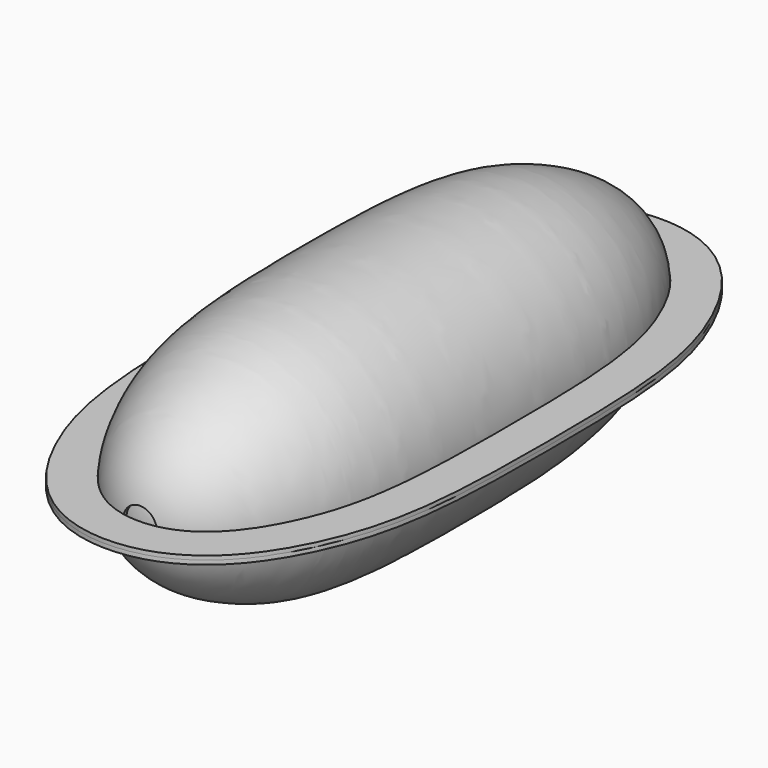
from build123d import *

# Parameters (mm, degrees)
F2_DEPTH = 1


# Not quite as in the source:
# - the dataset's text gives a spline's control points without its knots; the knots are read off the source's solid


with BuildPart() as f1:
    # F0 (on Top) → F1 (revolve)
    with BuildSketch(Plane.XY):
        with BuildLine():
            Line((-55.8199547231, 74.5623492029), (-56.5816092533, 75.4122275922))
            add(Edge.make_bspline(
                [(-56.5816092533, 75.4122275922), (-56.6397760093, 75.3978704726), (-58.3022178812, 74.9794709714), (-61.3612502345, 73.7570023616), (-65.2837059846, 71.035227187), (-68.6619012674, 67.6088358251), (-71.5492149944, 63.676466045), (-73.5896506783, 60.135000823), (-75.0264216479, 57.2332962118), (-76.0116188685, 55.0496489597), (-76.912177867, 52.8561250408), (-78.003679448, 49.8955719617), (-79.1717511063, 46.0950193349), (-80.2871106611, 41.2637042949), (-81.1460647488, 36.0501110723), (-81.9906513276, 28.4362571667), (-82.5604048188, 17.3855802508), (-82.6597137195, 6.2783429019), (-82.6597137195, 0)],
                knots=[0.0602391152, 0.0602391152, 0.0602391152, 0.0602391152, 0.0625, 0.125, 0.1875, 0.25, 0.3125, 0.375, 0.40625, 0.4375, 0.46875, 0.5, 0.5625, 0.625, 0.6875, 0.75, 0.875, 1, 1, 1, 1], degree=3))
            add(Edge.make_bspline(
                [(-55.8199547231, -75.5843198027), (-56.1355205763, -75.5195334393), (-58.0672567218, -75.0733675402), (-61.3612502345, -73.7570023616), (-65.2837059846, -71.035227187), (-68.6619012674, -67.6088358251), (-71.5492149944, -63.676466045), (-73.5896506783, -60.135000823), (-75.0264216479, -57.2332962118), (-76.0116188685, -55.0496489597), (-76.912177867, -52.8561250408), (-78.003679448, -49.8955719617), (-79.1717511063, -46.0950193349), (-80.2871106611, -41.2637042949), (-81.1460647488, -36.0501110723), (-81.9906513276, -28.4362571667), (-82.5604048188, -17.3855802508), (-82.6597137195, -6.2783429019), (-82.6597137195, 0)],
                knots=[0.0504643362, 0.0504643362, 0.0504643362, 0.0504643362, 0.0625, 0.125, 0.1875, 0.25, 0.3125, 0.375, 0.40625, 0.4375, 0.46875, 0.5, 0.5625, 0.625, 0.6875, 0.75, 0.875, 1, 1, 1, 1], degree=3))
            Line((-55.8199547231, -75.5843198027), (-55.8199547231, -74.5623492029))
            add(Edge.make_bspline(
                [(-55.8199547231, -74.5623492029), (-64.9610278539, -72.5808125911), (-79.9217070161, -51.0254234957), (-81.6597137195, -28.9947475074), (-81.6597137195, 0)],
                knots=[0.0531651237, 0.0531651237, 0.0531651237, 0.0531651237, 0.4222374323, 1, 1, 1, 1], degree=3))
            add(Edge.make_bspline(
                [(-55.8199547231, 74.5623492029), (-64.9610278539, 72.5808125911), (-79.9217070161, 51.0254234957), (-81.6597137195, 28.9947475074), (-81.6597137195, 0)],
                knots=[0.0531651237, 0.0531651237, 0.0531651237, 0.0531651237, 0.4222374323, 1, 1, 1, 1], degree=3))
        make_face()
    revolve(axis=Axis((-51.6597137195, -26.5565803749, 0), (0, -1, 0)))


with BuildPart() as f1b:
    # F0 (on Top) → F1, piece 2 (revolve)
    with BuildSketch(Plane.XY):
        with BuildLine():
            Line((-51.6597137195, -75), (-51.6597137195, 75))
            add(Edge.make_bspline(
                [(-51.6597137195, 75), (-53.117725446, 75), (-54.5031767561, 74.8477909354), (-55.8199547231, 74.5623492029)],
                knots=[0, 0, 0, 0, 0.0531651237, 0.0531651237, 0.0531651237, 0.0531651237], degree=3))
            Line((-55.8199547231, 74.5623492029), (-55.8199547231, -74.5623492029))
            add(Edge.make_bspline(
                [(-51.6597137195, -75), (-53.117725446, -75), (-54.5031767561, -74.8477909354), (-55.8199547231, -74.5623492029)],
                knots=[0, 0, 0, 0, 0.0531651237, 0.0531651237, 0.0531651237, 0.0531651237], degree=3))
        make_face()
    revolve(axis=Axis((-51.6597137195, -26.5565803749, 0), (0, -1, 0)))


with BuildPart() as f2:
    # F0 (on Top) → F2 (new body, symmetric)
    with BuildSketch(Plane.XY):
        with BuildLine():
            add(Edge.make_bspline(
                [(-51.6597137195, 76), (-53.3905810534, 76), (-55.0318116526, 75.794759317), (-56.5816092533, 75.4122275922)],
                knots=[0, 0, 0, 0, 0.0602391152, 0.0602391152, 0.0602391152, 0.0602391152], degree=3))
            add(Edge.make_bspline(
                [(-51.6597137195, 76), (-49.8638837493, 76), (-46.4652067363, 75.5581281718), (-41.9581772046, 73.7570023616), (-38.0357214545, 71.035227187), (-34.6575261717, 67.6088358251), (-31.7702124447, 63.676466045), (-29.7297767607, 60.135000823), (-28.2930057912, 57.2332962118), (-27.3078085706, 55.0496489597), (-26.407249572, 52.8561250408), (-25.3157479911, 49.8955719617), (-24.1476763328, 46.0950193349), (-23.0323167779, 41.2637042949), (-22.1733626903, 36.0501110723), (-21.3287761115, 28.4362571667), (-20.7590226202, 17.3855802508), (-20.6597137195, 6.2783429019), (-20.6597137195, 0)],
                knots=[0, 0, 0, 0, 0.0625, 0.125, 0.1875, 0.25, 0.3125, 0.375, 0.40625, 0.4375, 0.46875, 0.5, 0.5625, 0.625, 0.6875, 0.75, 0.875, 1, 1, 1, 1], degree=3))
            add(Edge.make_bspline(
                [(-51.6597137195, -76), (-49.8638837493, -76), (-46.4652067363, -75.5581281718), (-41.9581772046, -73.7570023616), (-38.0357214545, -71.035227187), (-34.6575261717, -67.6088358251), (-31.7702124447, -63.676466045), (-29.7297767607, -60.135000823), (-28.2930057912, -57.2332962118), (-27.3078085706, -55.0496489597), (-26.407249572, -52.8561250408), (-25.3157479911, -49.8955719617), (-24.1476763328, -46.0950193349), (-23.0323167779, -41.2637042949), (-22.1733626903, -36.0501110723), (-21.3287761115, -28.4362571667), (-20.7590226202, -17.3855802508), (-20.6597137195, -6.2783429019), (-20.6597137195, 0)],
                knots=[0, 0, 0, 0, 0.0625, 0.125, 0.1875, 0.25, 0.3125, 0.375, 0.40625, 0.4375, 0.46875, 0.5, 0.5625, 0.625, 0.6875, 0.75, 0.875, 1, 1, 1, 1], degree=3))
            Line((-51.6597137195, -76), (-51.6597137195, -86))
            add(Edge.make_bspline(
                [(-51.6597137195, -86), (-50.3517081027, -86), (-47.7690296636, -85.8387170423), (-44.0434614492, -85.1270052189), (-40.5305762875, -83.9819411512), (-37.2801784464, -82.4657547396), (-34.314441056, -80.6466412752), (-30.747422832, -77.9115906547), (-27.7293267494, -74.8335900569), (-25.1628486092, -71.5853173338), (-23.4375735308, -69.0912636735), (-21.889348579, -66.5656635825), (-20.4969514445, -64.0265948028), (-19.2486638728, -61.504363593), (-18.1227411236, -59.0086196482), (-17.0880446352, -56.4887914009), (-15.8261069566, -53.0664581165), (-14.4779141554, -48.6774501047), (-13.2101618031, -43.1772674245), (-12.2581535204, -37.384955502), (-11.3474379426, -29.1494372612), (-10.7592725159, -17.6080481383), (-10.6597137195, -6.3310685453), (-10.6597137195, 0)],
                knots=[0, 0, 0, 0, 0.03125, 0.0625, 0.09375, 0.125, 0.15625, 0.1875, 0.25, 0.28125, 0.3125, 0.34375, 0.375, 0.40625, 0.4375, 0.46875, 0.5, 0.5625, 0.625, 0.6875, 0.75, 0.875, 1, 1, 1, 1], degree=3))
            add(Edge.make_bspline(
                [(-51.6597137195, 86), (-50.3517081027, 86), (-47.7690296636, 85.8387170423), (-44.0434614492, 85.1270052189), (-40.5305762875, 83.9819411512), (-37.2801784464, 82.4657547396), (-34.314441056, 80.6466412752), (-30.747422832, 77.9115906547), (-27.7293267494, 74.8335900569), (-25.1628486092, 71.5853173338), (-23.4375735308, 69.0912636735), (-21.889348579, 66.5656635825), (-20.4969514445, 64.0265948028), (-19.2486638728, 61.504363593), (-18.1227411236, 59.0086196482), (-17.0880446352, 56.4887914009), (-15.8261069566, 53.0664581165), (-14.4779141554, 48.6774501047), (-13.2101618031, 43.1772674245), (-12.2581535204, 37.384955502), (-11.3474379426, 29.1494372612), (-10.7592725159, 17.6080481383), (-10.6597137195, 6.3310685453), (-10.6597137195, 0)],
                knots=[0, 0, 0, 0, 0.03125, 0.0625, 0.09375, 0.125, 0.15625, 0.1875, 0.25, 0.28125, 0.3125, 0.34375, 0.375, 0.40625, 0.4375, 0.46875, 0.5, 0.5625, 0.625, 0.6875, 0.75, 0.875, 1, 1, 1, 1], degree=3))
            add(Edge.make_bspline(
                [(-51.6597137195, 86), (-52.9677193364, 86), (-55.5503977755, 85.8387170423), (-59.2759659899, 85.1270052189), (-61.9911504677, 84.2419605791), (-63.4592895327, 83.6310316869), (-63.8095950817, 83.4774444461)],
                knots=[0, 0, 0, 0, 0.03125, 0.0625, 0.09375, 0.1037113909, 0.1037113909, 0.1037113909, 0.1037113909], degree=3))
            Line((-63.8095950817, 83.4774444461), (-56.5816092533, 75.4122275922))
        make_face()
        with BuildLine():
            add(Edge.make_bspline(
                [(-56.5816092533, 75.4122275922), (-56.6397760093, 75.3978704726), (-58.3022178812, 74.9794709714), (-61.3612502345, 73.7570023616), (-65.2837059846, 71.035227187), (-68.6619012674, 67.6088358251), (-71.5492149944, 63.676466045), (-73.5896506783, 60.135000823), (-75.0264216479, 57.2332962118), (-76.0116188685, 55.0496489597), (-76.912177867, 52.8561250408), (-78.003679448, 49.8955719617), (-79.1717511063, 46.0950193349), (-80.2871106611, 41.2637042949), (-81.1460647488, 36.0501110723), (-81.9906513276, 28.4362571667), (-82.5604048188, 17.3855802508), (-82.6597137195, 6.2783429019), (-82.6597137195, 0)],
                knots=[0.0602391152, 0.0602391152, 0.0602391152, 0.0602391152, 0.0625, 0.125, 0.1875, 0.25, 0.3125, 0.375, 0.40625, 0.4375, 0.46875, 0.5, 0.5625, 0.625, 0.6875, 0.75, 0.875, 1, 1, 1, 1], degree=3))
            Line((-56.5816092533, 75.4122275922), (-63.8095950817, 83.4774444461))
            add(Edge.make_bspline(
                [(-63.8095950817, 83.4774444461), (-64.5582373144, 83.149211293), (-66.3543729327, 82.2724651368), (-69.0049863831, 80.6466412752), (-72.572004607, 77.9115906547), (-75.5901006897, 74.8335900569), (-78.1565788298, 71.5853173338), (-79.8818539083, 69.0912636735), (-81.4300788601, 66.5656635825), (-82.8224759946, 64.0265948028), (-84.0707635663, 61.504363593), (-85.1966863154, 59.0086196482), (-86.2313828039, 56.4887914009), (-87.4933204824, 53.0664581165), (-88.8415132837, 48.6774501047), (-90.109265636, 43.1772674245), (-91.0612739187, 37.384955502), (-91.9719894964, 29.1494372612), (-92.5601549232, 17.6080481383), (-92.6597137195, 6.3310685453), (-92.6597137195, 0)],
                knots=[0.1037113909, 0.1037113909, 0.1037113909, 0.1037113909, 0.125, 0.15625, 0.1875, 0.25, 0.28125, 0.3125, 0.34375, 0.375, 0.40625, 0.4375, 0.46875, 0.5, 0.5625, 0.625, 0.6875, 0.75, 0.875, 1, 1, 1, 1], degree=3))
            add(Edge.make_bspline(
                [(-51.6597137195, -86), (-52.9677193364, -86), (-55.5503977755, -85.8387170423), (-59.2759659899, -85.1270052189), (-62.7888511515, -83.9819411512), (-66.0392489927, -82.4657547396), (-69.0049863831, -80.6466412752), (-72.572004607, -77.9115906547), (-75.5901006897, -74.8335900569), (-78.1565788298, -71.5853173338), (-79.8818539083, -69.0912636735), (-81.4300788601, -66.5656635825), (-82.8224759946, -64.0265948028), (-84.0707635663, -61.504363593), (-85.1966863154, -59.0086196482), (-86.2313828039, -56.4887914009), (-87.4933204824, -53.0664581165), (-88.8415132837, -48.6774501047), (-90.109265636, -43.1772674245), (-91.0612739187, -37.384955502), (-91.9719894964, -29.1494372612), (-92.5601549232, -17.6080481383), (-92.6597137195, -6.3310685453), (-92.6597137195, 0)],
                knots=[0, 0, 0, 0, 0.03125, 0.0625, 0.09375, 0.125, 0.15625, 0.1875, 0.25, 0.28125, 0.3125, 0.34375, 0.375, 0.40625, 0.4375, 0.46875, 0.5, 0.5625, 0.625, 0.6875, 0.75, 0.875, 1, 1, 1, 1], degree=3))
            Line((-51.6597137195, -86), (-51.6597137195, -76))
            add(Edge.make_bspline(
                [(-51.6597137195, -76), (-53.1097195977, -76), (-54.4968186185, -75.8559625536), (-55.8199547231, -75.5843198027)],
                knots=[0, 0, 0, 0, 0.0504643362, 0.0504643362, 0.0504643362, 0.0504643362], degree=3))
            add(Edge.make_bspline(
                [(-55.8199547231, -75.5843198027), (-56.1355205763, -75.5195334393), (-58.0672567218, -75.0733675402), (-61.3612502345, -73.7570023616), (-65.2837059846, -71.035227187), (-68.6619012674, -67.6088358251), (-71.5492149944, -63.676466045), (-73.5896506783, -60.135000823), (-75.0264216479, -57.2332962118), (-76.0116188685, -55.0496489597), (-76.912177867, -52.8561250408), (-78.003679448, -49.8955719617), (-79.1717511063, -46.0950193349), (-80.2871106611, -41.2637042949), (-81.1460647488, -36.0501110723), (-81.9906513276, -28.4362571667), (-82.5604048188, -17.3855802508), (-82.6597137195, -6.2783429019), (-82.6597137195, 0)],
                knots=[0.0504643362, 0.0504643362, 0.0504643362, 0.0504643362, 0.0625, 0.125, 0.1875, 0.25, 0.3125, 0.375, 0.40625, 0.4375, 0.46875, 0.5, 0.5625, 0.625, 0.6875, 0.75, 0.875, 1, 1, 1, 1], degree=3))
        make_face()
    extrude(amount=F2_DEPTH, both=True)


solid = Compound([f1.part, f1b.part, f2.part])
